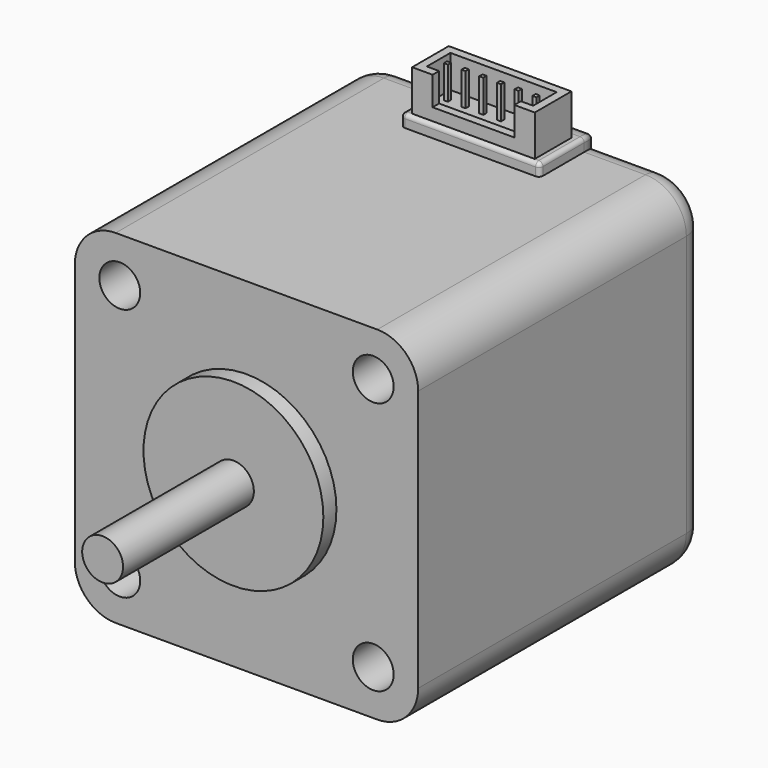
from build123d import *

# Parameters (mm, degrees)
F0_W      = 42
F0_H      = 42
F1_DEPTH  = 44
F2_R      = 11
F3_DEPTH  = 2
F4_R      = 2.5
F5_DEPTH  = 20
F6_R      = 2.5
F7_DEPTH  = 10
F8_W      = 17
F8_H      = 9.8
F9_DEPTH  = 1.5
F10_R     = 5
F11_R     = 3
F12_W     = 15
F12_H     = 5.6
F13_DEPTH = 1
F14_W     = 15
F14_H     = 5.6
F14_W_2   = 13
F14_H_2   = 3.6
F15_DEPTH = 4
F16_W     = 0.5
F16_H     = 0.5
F17_DEPTH = 4
F18_R     = 0.49999
F19_W     = 10
F19_H     = 1
F20_DEPTH = 3.5


# Not quite as in the source:
# - a fillet or chamfer is up to 0.001 mm smaller than in the source, because OpenCascade refuses the exact size


with BuildPart() as f1:
    # F0 (on Front) → F1 (new body)
    with BuildSketch(Plane.XZ):
        Rectangle(F0_W, F0_H)
    extrude(amount=F1_DEPTH)

    # F2 (on face) → F3 (join)
    with BuildSketch(Plane.XZ.offset(44)):
        Circle(F2_R)
    extrude(amount=F3_DEPTH)

    # F4 (on face) → F5 (join)
    with BuildSketch(Plane.XZ.offset(46)):
        Circle(F4_R)
    extrude(amount=F5_DEPTH)

    # F6 (on face) → F7 (cut)
    with BuildSketch(Plane.XZ.offset(44)):
        with Locations((-15.5, 15.5)):
            Circle(F6_R)
        with Locations((15.5, 15.5)):
            Circle(F6_R)
        with Locations((15.5, -15.5)):
            Circle(F6_R)
        with Locations((-15.5, -15.5)):
            Circle(F6_R)
    extrude(amount=-F7_DEPTH, mode=Mode.SUBTRACT)

    # F8 (on face) → F9 (join)
    with BuildSketch(Plane.XY.offset(21)):
        with Locations((0, -4.9)):
            Rectangle(F8_W, F8_H)
    extrude(amount=F9_DEPTH)

    # F10
    f10_edges = [f1.edges().sort_by_distance(p)[0] for p in [
        (-21, -22, 21),
        (21, -22, 21),
        (21, -22, -21),
        (-21, -22, -21),
    ]]
    fillet(f10_edges, radius=F10_R)

    # F11
    f11_edges = [f1.edges().sort_by_distance(p)[0] for p in [
        (12.25, 0, 21),
        (19.535534, 0, 19.535534),
        (8.5, 0, 21.75),
        (21, 0, 0),
        (0, 0, 22.5),
        (19.535534, 0, -19.535534),
        (-8.5, 0, 21.75),
        (0, 0, -21),
        (-12.25, 0, 21),
        (-19.535534, 0, -19.535534),
        (-19.535534, 0, 19.535534),
        (-21, 0, 0),
    ]]
    fillet(f11_edges, radius=F11_R)

    # F12 (on face) → F13 (join)
    with BuildSketch(Plane.XY.offset(22.5)):
        with Locations((0, -6.5)):
            Rectangle(F12_W, F12_H)
    extrude(amount=F13_DEPTH)

    # F14 (on face) → F15 (join)
    with BuildSketch(Plane.XY.offset(23.5)):
        with Locations((0, -6.5)):
            Rectangle(F14_W, F14_H)
        with Locations((0, -6.5)):
            Rectangle(F14_W_2, F14_H_2, mode=Mode.SUBTRACT)
    extrude(amount=F15_DEPTH)

    # F16 (on face) → F17 (join)
    with BuildSketch(Plane.XY.offset(23.5)):
        with Locations((-5.417, -6.5)):
            Rectangle(F16_W, F16_H)
        with Locations((-3.25, -6.5)):
            Rectangle(F16_W, F16_H)
        with Locations((-1.083, -6.5)):
            Rectangle(F16_W, F16_H)
        with Locations((3.25, -6.5)):
            Rectangle(F16_W, F16_H)
        with Locations((1.083, -6.5)):
            Rectangle(F16_W, F16_H)
        with Locations((5.417, -6.5)):
            Rectangle(F16_W, F16_H)
    extrude(amount=F17_DEPTH)

    # F18 (radius 0.5 in the source; OpenCascade refuses exactly that, so slightly less here)
    f18_edges = [f1.edges().sort_by_distance(p)[0] for p in [
        (0, -9.8, 22.5),
        (8.5, -9.8, 21.75),
        (8.5, -6.4, 22.5),
        (-8.5, -9.8, 21.75),
        (-8.5, -6.4, 22.5),
        (-7.438147, -0.710112, 21.438147),
        (7.438147, -0.710112, 21.438147),
        (0, 0, 19.5),
        (5.5, 0, 18.75),
        (-5.5, 0, 18.75),
    ]]
    fillet(f18_edges, radius=F18_R)

    # F19 (on face) → F20 (cut)
    with BuildSketch(Plane.XY.offset(27.5)):
        with Locations((0, -8.8)):
            Rectangle(F19_W, F19_H)
    extrude(amount=-F20_DEPTH, mode=Mode.SUBTRACT)


solid = f1.part
